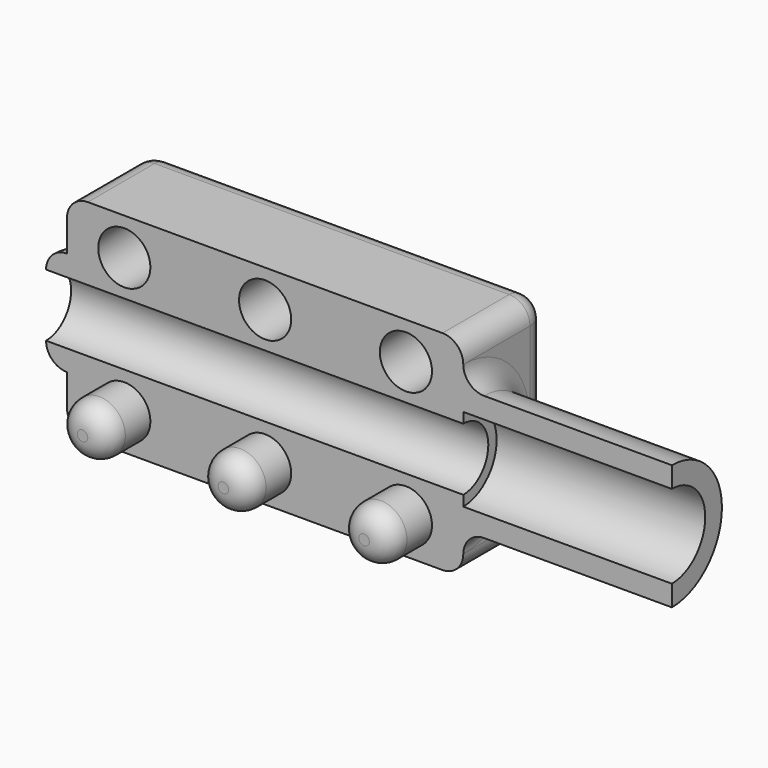
from build123d import *

# Parameters (mm, degrees)
F1_ANGLE = 180
F2_W     = 19
F2_H     = 10
F3_DEPTH = 5
F4_R     = 1.5
F5_DEPTH = 25
F6_R     = 1.25
F7_DEPTH = 2.5
F8_DEPTH = 2.5
F9_R     = 0.99999
F10_R    = 0.99999
F11_R    = 1
F11_2_R  = 1
F11_3_R  = 1


# Not quite as in the source:
# - a fillet or chamfer is up to 0.001 mm smaller than in the source, because OpenCascade refuses the exact size


with BuildPart() as f1:
    # F0 (on Front) → F1 (revolve)
    with BuildSketch(Plane.XZ):
        Polygon((-5, 2), (5, 2), (5, 3), (-5.9999994636, 3), (-6, 2.5), (-25, 2.5), (-25, 1.5), (-5, 1.5), align=None)
    revolve(axis=Axis((-10, 0, 0), (-1, 0, 0)), revolution_arc=F1_ANGLE)

    # F2 (on Front) → F3 (join)
    with BuildSketch(Plane.XZ):
        with Locations((-14.5, 0)):
            Rectangle(F2_W, F2_H)
    extrude(amount=-F3_DEPTH)

    # F4 (on Right) → F5 (cut)
    with BuildSketch(Plane.YZ):
        Circle(F4_R)
    extrude(amount=-F5_DEPTH, mode=Mode.SUBTRACT)

    # F6 (on Front) → F7 (cut)
    with BuildSketch(Plane.XZ):
        with Locations((-21.25, 3.2196251888)):
            Circle(F6_R)
        with Locations((-14.5, 3.2196251888)):
            Circle(F6_R)
        with Locations((-7.75, 3.2196251888)):
            Circle(F6_R)
    extrude(amount=-F7_DEPTH, mode=Mode.SUBTRACT)

    # F9 (radius 1 in the source; OpenCascade refuses exactly that, so slightly less here)
    f9_edges = [f1.edges().sort_by_distance(p)[0] for p in [
        (-5, 2.5, 5),
        (-14.5, 5, 5),
        (-5, 5, 0),
        (-24, 5, 0),
        (-24, 2.5, 5),
        (-24, 2.5, -5),
        (-14.5, 5, -5),
        (-5, 2.5, -5),
        (-5, 3, 0),
    ]]
    fillet(f9_edges, radius=F9_R)

    # F10 (radius 1 in the source; OpenCascade refuses exactly that, so slightly less here)
    f10_edges = [f1.edges().sort_by_distance(p)[0] for p in [
        (-25, 2.5, 0),
    ]]
    fillet(f10_edges, radius=F10_R)


with BuildPart() as f8:
    # F6 (on Front) → F8 (new body)
    with BuildSketch(Plane.XZ):
        with Locations((-21.25, -3.2803748112)):
            Circle(F6_R)
    extrude(amount=F8_DEPTH)

    # F11
    f11_edges = [f8.edges().sort_by_distance(p)[0] for p in [
        (-22.5, -2.5, -3.280375),
    ]]
    fillet(f11_edges, radius=F11_R)


with BuildPart() as f8b:
    # F6 (on Front) → F8, piece 2 (new body)
    with BuildSketch(Plane.XZ):
        with Locations((-14.5, -3.2803748112)):
            Circle(F6_R)
    extrude(amount=F8_DEPTH)

    # F11#2
    f11_2_edges = [f8b.edges().sort_by_distance(p)[0] for p in [
        (-15.75, -2.5, -3.280375),
    ]]
    fillet(f11_2_edges, radius=F11_2_R)


with BuildPart() as f8c:
    # F6 (on Front) → F8, piece 3 (new body)
    with BuildSketch(Plane.XZ):
        with Locations((-7.75, -3.2803748112)):
            Circle(F6_R)
    extrude(amount=F8_DEPTH)

    # F11#3
    f11_3_edges = [f8c.edges().sort_by_distance(p)[0] for p in [
        (-9, -2.5, -3.280375),
    ]]
    fillet(f11_3_edges, radius=F11_3_R)


solid = Compound([f1.part, f8.part, f8b.part, f8c.part])
